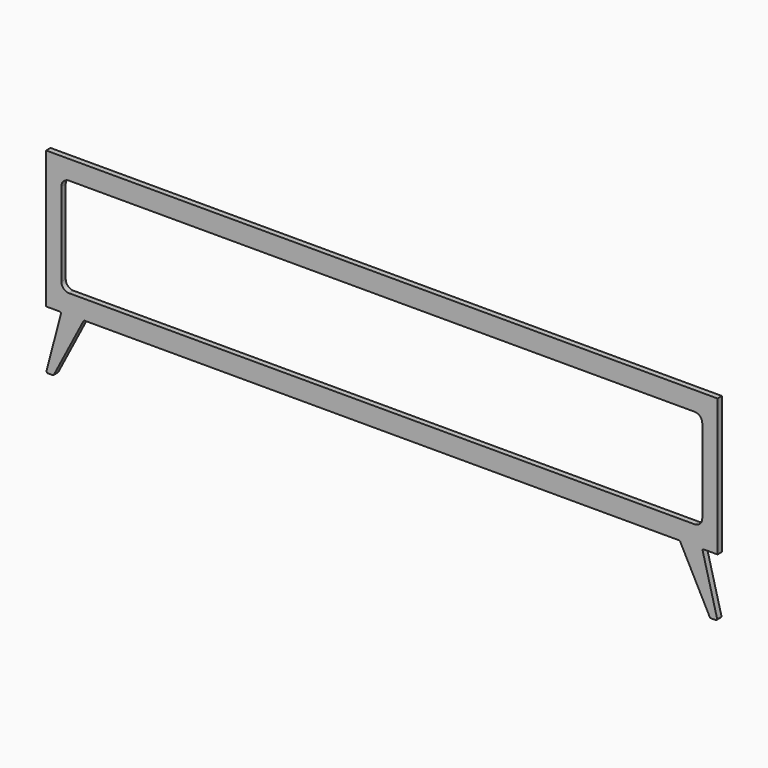
from build123d import *

# Parameters (mm, degrees)
F0_W     = 9
F0_H     = 9
F0_H_2   = 432
F1_DEPTH = 18


# Not quite as in the source:
# - a feature names something its author has since deleted; it is built from what else it names


with BuildPart() as f1:
    # F0 (on Front) → F1 (new body)
    with BuildSketch(Plane.XZ):
        with Locations((-1095.5, 71.3756743552)):
            Rectangle(F0_W, F0_H)
        with BuildLine():
            Line((-973.3476458471, -374.1243256448), (-1054.6076226562, -374.1243256448))
            ThreePointArc((-1054.6076226562, -374.1243256448), (-1051.7483407187, -375.721921149), (-1051.265639742, -378.9614896944))
            Line((-1051.265639742, -378.9614896944), (-1098.3606008427, -558.954299013))
            ThreePointArc((-1098.3606008427, -558.954299013), (-1097.4812264988, -563.2754093644), (-1093.523436793, -565.219938755))
            Line((-1093.523436793, -565.219938755), (-1078.8076104242, -565.219938755))
            ThreePointArc((-1078.8076104242, -565.219938755), (-1076.2129629213, -564.4940239596), (-1074.371712623, -562.5270604893))
            Line((-1074.371712623, -562.5270604893), (-977.7835436484, -376.8172039105))
            ThreePointArc((-977.7835436484, -376.8172039105), (-975.94229335, -374.8502404402), (-973.3476458471, -374.1243256448))
        make_face()
        with BuildLine():
            Line((0, -365.1243256448), (-1091, -365.1243256448))
            Line((-1091, -365.1243256448), (-1091, -374.1243256448))
            Line((-1091, -374.1243256448), (-1055, -374.1243256448))
            ThreePointArc((-1055, -374.1243256448), (-1054.8038113281, -374.1191399972), (-1054.6076226562, -374.1243256448))
            Line((-1054.6076226562, -374.1243256448), (-973.3476458471, -374.1243256448))
            Line((-973.3476458471, -374.1243256448), (0, -374.1243256448))
            Line((0, -374.1243256448), (973.3476458471, -374.1243256448))
            Line((973.3476458471, -374.1243256448), (1054.6076226562, -374.1243256448))
            ThreePointArc((1054.6076226562, -374.1243256448), (1054.8038113281, -374.1191399972), (1055, -374.1243256448))
            Line((1055, -374.1243256448), (1100, -374.1243256448))
            Line((1100, -374.1243256448), (1100, 66.8756743552))
            Line((1100, 66.8756743552), (1091, 66.8756743552))
            Line((1091, 66.8756743552), (1091, -365.0378882885))
            Line((1091, -365.0378882885), (1091, -365.1243256448))
            Line((1091, -365.1243256448), (0, -365.1243256448))
        make_face()
        Polygon((0, 75.8756743552), (-1091, 75.8756743552), (-1091, 66.8756743552), (0, 66.8756743552), (1091, 66.8756743552), (1091, 75.8756743552), align=None)
        with Locations((-1095.5, -149.1243256448)):
            Rectangle(F0_W, F0_H_2)
        with Locations((-1095.5, -369.6243256448)):
            Rectangle(F0_W, F0_H)
        with Locations((1095.5, 71.3756743552)):
            Rectangle(F0_W, F0_H)
        with BuildLine():
            ThreePointArc((1051.265639742, -378.9614896944), (1051.7483407187, -375.721921149), (1054.6076226562, -374.1243256448))
            Line((1054.6076226562, -374.1243256448), (973.3476458471, -374.1243256448))
            ThreePointArc((973.3476458471, -374.1243256448), (975.94229335, -374.8502404402), (977.7835436484, -376.8172039105))
            Line((977.7835436484, -376.8172039105), (1074.371712623, -562.5270604893))
            ThreePointArc((1074.371712623, -562.5270604893), (1076.2129629213, -564.4940239596), (1078.8076104242, -565.219938755))
            Line((1078.8076104242, -565.219938755), (1093.523436793, -565.219938755))
            ThreePointArc((1093.523436793, -565.219938755), (1097.4812264988, -563.2754093644), (1098.3606008427, -558.954299013))
            Line((1098.3606008427, -558.954299013), (1051.265639742, -378.9614896944))
        make_face()
        Polygon((0, 66.8756743552), (-1091, 66.8756743552), (-1091, -365.1243256448), (0, -365.1243256448), (1091, -365.1243256448), (1091, -365.0378882885), (1091, 66.8756743552), align=None)
        with BuildLine():
            Line((-1049.9993757457, -21.1739316583), (-1049.9993757457, -21.1230870336))
            Line((-1049.9993757457, -21.1230870336), (-1049.9993757457, -11.824025))
            ThreePointArc((-1049.9993757457, -11.824025), (-1042.6770452754, 5.8536445296), (-1024.9993757457, 13.175975))
            Line((-1024.9993757457, 13.175975), (1024.9993757457, 13.175975))
            ThreePointArc((1024.9993757457, 13.175975), (1042.6770452754, 5.8536445296), (1049.9993757457, -11.824025))
            Line((1049.9993757457, -11.824025), (1049.9993757457, -286.3619962875))
            ThreePointArc((1049.9993757457, -286.3619962875), (1042.6770452754, -304.0396658171), (1024.9993757457, -311.3619962875))
            Line((1024.9993757457, -311.3619962875), (-1024.9993757457, -311.3619962875))
            ThreePointArc((-1024.9993757457, -311.3619962875), (-1042.6770452754, -304.0396658171), (-1049.9993757457, -286.3619962875))
            Line((-1049.9993757457, -286.3619962875), (-1049.9993757457, -21.1739316583))
        make_face(mode=Mode.SUBTRACT)
    extrude(amount=F1_DEPTH)


solid = f1.part
